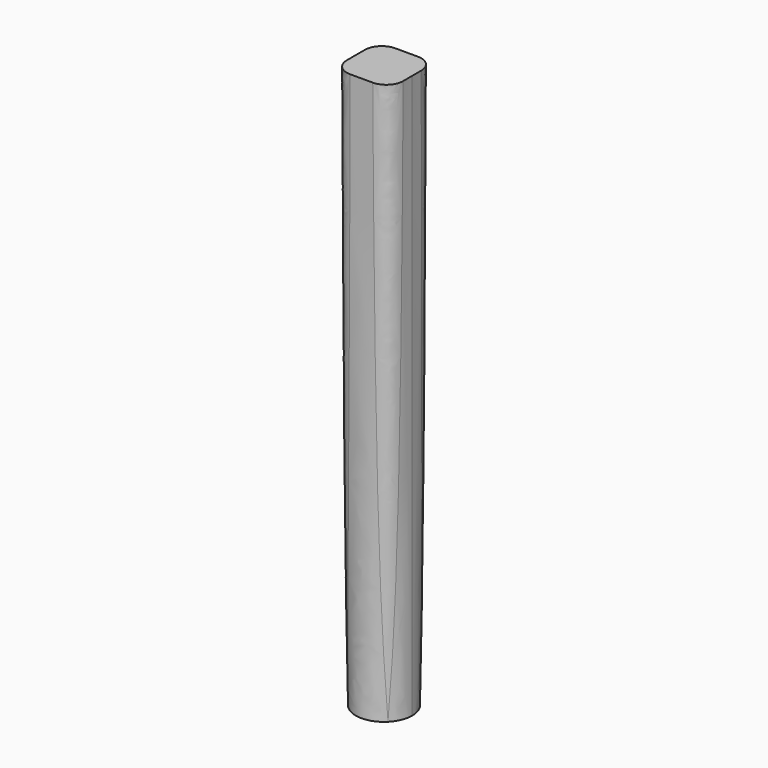
from build123d import *

# Parameters (mm, degrees)
F0_R = 25
F2_W = 50
F2_H = 50
F4_R = 15


with BuildPart() as f3:
    # F0 (on Top) → F3 section 0
    with BuildSketch(Plane.XY):
        Circle(F0_R)
    # F2 (on offset) → F3 section 1
    with BuildSketch(Plane.XY.offset(500)):
        Rectangle(F2_W, F2_H)
    loft()

    # F4
    f4_edges = [f3.edges().sort_by_distance(p)[0] for p in [
        (21.338835, 21.338835, 250),
        (-21.338835, 21.338835, 250),
        (-21.338835, -21.338835, 250),
        (21.338835, -21.338835, 250),
    ]]
    fillet(f4_edges, radius=F4_R)


solid = f3.part
